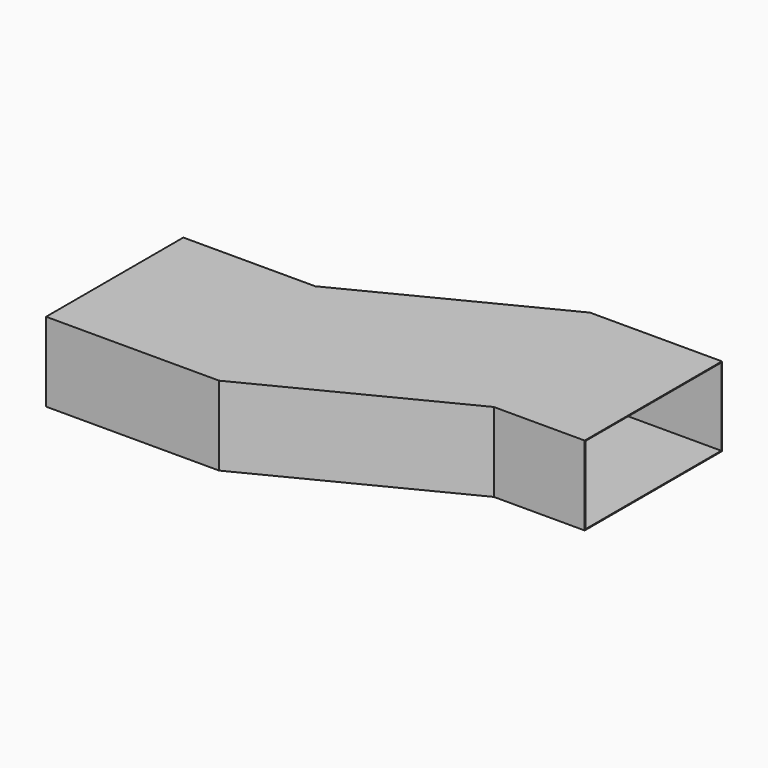
from build123d import *

# Parameters (mm, degrees)
F1_DEPTH = 300
F2_T     = -3


with BuildPart() as f1:
    # F0 (on Top) → F1 (new body)
    with BuildSketch(Plane.XY):
        Polygon((0, 650), (0, 0), (655.664250573, 0), (1395.664250573, 376), (1740, 376), (1740, 1026), (1240, 1026), (500, 650), align=None)
    extrude(amount=F1_DEPTH)

    # F2
    f2_openings = [f1.faces().sort_by_distance(p)[0] for p in [
        (0, 325, 150),
        (1740, 701, 150),
    ]]
    offset(amount=F2_T, openings=f2_openings, kind=Kind.INTERSECTION)


solid = f1.part
